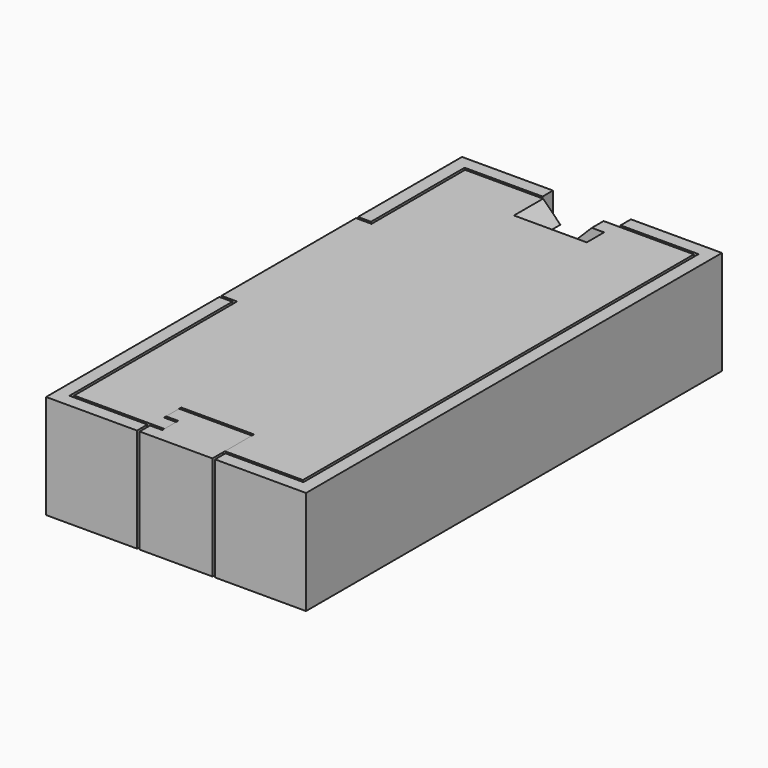
from build123d import *

# Parameters (mm, degrees)
F0_W      = 30
F0_H      = 60
F0_W_2    = 27
F0_H_2    = 57
F0_W_3    = 26.4
F0_H_3    = 56.4
F0_W_4    = 24
F0_H_4    = 54
F1_DEPTH  = 10
F2_DEPTH  = 3
F3_W      = 30
F3_H      = 60
F4_DEPTH  = 2
F6_DEPTH  = 24
F7_DEPTH  = 2
F10_DEPTH = 1.8
F11_DEPTH = 6
F12_START = -3.5
F12_DEPTH = 2.5
F14_DEPTH = 1.8
F15_DEPTH = 6
F16_START = -3.5
F16_DEPTH = 2.5
F17_DEPTH = 6
F18_START = -3.5
F18_DEPTH = 2.5
F19_W     = 8.4
F19_H     = 12
F20_DEPTH = 1.5
F21_DEPTH = 5.7
F22_START = -3.8
F22_DEPTH = 1.9
F23_DEPTH = 6
F24_START = -3.5
F24_DEPTH = 2.5
F25_W     = 20
F25_H     = 8
F26_DEPTH = 3
F27_W     = 3
F27_H     = 19.4
F28_DEPTH = 4
F30_DEPTH = 4.2


with BuildPart() as f1:
    # F0 (on Top) → F1 (new body)
    with BuildSketch(Plane.XY):
        with Locations((15, 30)):
            Rectangle(F0_W, F0_H)
        with Locations((15, 30)):
            Rectangle(F0_W_2, F0_H_2, mode=Mode.SUBTRACT)
        with Locations((15, 30)):
            Rectangle(F0_W_2, F0_H_2)
        with Locations((15, 30)):
            Rectangle(F0_W_3, F0_H_3, mode=Mode.SUBTRACT)
        with Locations((15, 30)):
            Rectangle(F0_W_3, F0_H_3)
        with Locations((15, 30)):
            Rectangle(F0_W_4, F0_H_4, mode=Mode.SUBTRACT)
    extrude(amount=-F1_DEPTH)

    # F0 (on Top) → F2 (cut)
    with BuildSketch(Plane.XY):
        with Locations((15, 30)):
            Rectangle(F0_W_2, F0_H_2)
        with Locations((15, 30)):
            Rectangle(F0_W_3, F0_H_3, mode=Mode.SUBTRACT)
        with Locations((15, 30)):
            Rectangle(F0_W_3, F0_H_3)
        with Locations((15, 30)):
            Rectangle(F0_W_4, F0_H_4, mode=Mode.SUBTRACT)
    extrude(amount=-F2_DEPTH, mode=Mode.SUBTRACT)

    # F3 (on face) → F4 (join)
    with BuildSketch(Plane(origin=(0, 0, -10), x_dir=(1, 0, 0), z_dir=(0, 0, -1))):
        with Locations((15, -30)):
            Rectangle(F3_W, F3_H)
    extrude(amount=F4_DEPTH)

    # F5 (on face) → F6 (join, through all)
    with BuildSketch(Plane(origin=(27, 0, 0), x_dir=(0, -1, 0), z_dir=(-1, 0, 0))):
        Polygon((-8, -5), (-3, -10), (-3, -5), align=None)
        Polygon((-57, -5), (-57, -10), (-52, -5), align=None)
    extrude(amount=F6_DEPTH)

    # F9 (on face) → F10 (cut, through all)
    with BuildSketch(Plane.XZ):
        Polygon((10.8, 0), (10.5, 0), (10.5, -12), (10.8, -12), (15, -7.8), (15.7071067812, -8.5071067812), (19.2, -12), (19.5, -12), (19.5, 0), (19.2, 0), (17.2, -2), (14.2142135624, -2), (12.8, -2), align=None)
        Polygon((12.2142135624, 0), (10.8, 0), (12.8, -2), (14.2142135624, -2), align=None)
        Polygon((19.2, 0), (12.2142135624, 0), (14.2142135624, -2), (17.2, -2), align=None)
        Polygon((15.7071067812, -8.5071067812), (12.2142135624, -12), (19.2, -12), align=None)
        Polygon((15, -7.8), (10.8, -12), (12.2142135624, -12), (15.7071067812, -8.5071067812), align=None)
    extrude(amount=-F10_DEPTH, mode=Mode.SUBTRACT)

    # F13 (on face) → F14 (cut, through all)
    with BuildSketch(Plane(origin=(0, 60, 0), x_dir=(-1, 0, 0), z_dir=(0, 1, 0))):
        Polygon((-19.2, 0), (-19.5, 0), (-19.5, -12), (-19.2, -12), (-15, -7.8), (-14.2928932188, -8.5071067812), (-10.8, -12), (-10.5, -12), (-10.5, 0), (-10.8, 0), (-12.8, -2), (-15.7857864376, -2), (-17.2, -2), align=None)
        Polygon((-17.7857864376, 0), (-19.2, 0), (-17.2, -2), (-15.7857864376, -2), align=None)
        Polygon((-10.8, 0), (-17.7857864376, 0), (-15.7857864376, -2), (-12.8, -2), align=None)
        Polygon((-14.2928932188, -8.5071067812), (-17.7857864376, -12), (-10.8, -12), align=None)
        Polygon((-15, -7.8), (-19.2, -12), (-17.7857864376, -12), (-14.2928932188, -8.5071067812), align=None)
    extrude(amount=-F14_DEPTH, mode=Mode.SUBTRACT)

    # F9 (on face) → F17 (cut)
    with BuildSketch(Plane.XZ):
        Polygon((15.7071067812, -8.5071067812), (12.2142135624, -12), (19.2, -12), align=None)
    extrude(amount=-F17_DEPTH, mode=Mode.SUBTRACT)

    # F9 (on face) → F18 (cut)
    with BuildSketch(Plane.XZ.offset(F18_START)):
        Polygon((15, -7.8), (10.8, -12), (12.2142135624, -12), (15.7071067812, -8.5071067812), align=None)
    extrude(amount=-F18_DEPTH, mode=Mode.SUBTRACT)

    # F13 (on face) → F23 (cut)
    with BuildSketch(Plane(origin=(0, 60, 0), x_dir=(-1, 0, 0), z_dir=(0, 1, 0))):
        Polygon((-14.2928932188, -8.5071067812), (-17.7857864376, -12), (-10.8, -12), align=None)
    extrude(amount=-F23_DEPTH, mode=Mode.SUBTRACT)

    # F13 (on face) → F24 (cut)
    with BuildSketch(Plane(origin=(0, 60, 0), x_dir=(-1, 0, 0), z_dir=(0, 1, 0)).offset(F24_START)):
        Polygon((-15, -7.8), (-19.2, -12), (-17.7857864376, -12), (-14.2928932188, -8.5071067812), align=None)
    extrude(amount=-F24_DEPTH, mode=Mode.SUBTRACT)

    # F25 (on face) → F26 (cut, through all)
    with BuildSketch(Plane(origin=(0, 0, 0), x_dir=(0, -1, 0), z_dir=(-1, 0, 0))):
        with Locations((-35, -4)):
            Rectangle(F25_W, F25_H)
    extrude(amount=-F26_DEPTH, mode=Mode.SUBTRACT)


with BuildPart() as f7:
    # F0 (on Top) → F7 (new body)
    with BuildSketch(Plane.XY):
        with Locations((15, 30)):
            Rectangle(F0_W_3, F0_H_3)
        with Locations((15, 30)):
            Rectangle(F0_W_4, F0_H_4, mode=Mode.SUBTRACT)
        with Locations((15, 30)):
            Rectangle(F0_W_4, F0_H_4)
    extrude(amount=-F7_DEPTH)

    # F9 (on face) → F11 (cut)
    with BuildSketch(Plane.XZ):
        Polygon((19.2, 0), (12.2142135624, 0), (14.2142135624, -2), (17.2, -2), align=None)
    extrude(amount=-F11_DEPTH, mode=Mode.SUBTRACT)

    # F9 (on face) → F12 (cut)
    with BuildSketch(Plane.XZ.offset(F12_START)):
        Polygon((12.2142135624, 0), (10.8, 0), (12.8, -2), (14.2142135624, -2), align=None)
    extrude(amount=-F12_DEPTH, mode=Mode.SUBTRACT)

    # F13 (on face) → F15 (cut)
    with BuildSketch(Plane(origin=(0, 60, 0), x_dir=(-1, 0, 0), z_dir=(0, 1, 0))):
        Polygon((-10.8, 0), (-17.7857864376, 0), (-15.7857864376, -2), (-12.8, -2), align=None)
    extrude(amount=-F15_DEPTH, mode=Mode.SUBTRACT)

    # F13 (on face) → F16 (cut)
    with BuildSketch(Plane(origin=(0, 60, 0), x_dir=(-1, 0, 0), z_dir=(0, 1, 0)).offset(F16_START)):
        Polygon((-17.7857864376, 0), (-19.2, 0), (-17.2, -2), (-15.7857864376, -2), align=None)
    extrude(amount=-F16_DEPTH, mode=Mode.SUBTRACT)

    # F27 (on face) → F28 (join)
    with BuildSketch(Plane.XY):
        with Locations((1.5, 35)):
            Rectangle(F27_W, F27_H)
    extrude(amount=-F28_DEPTH)


with BuildPart() as f20:
    # F19 (on face) → F20 (new body)
    with BuildSketch(Plane.XZ):
        with Locations((15, -6)):
            Rectangle(F19_W, F19_H)
    extrude(amount=-F20_DEPTH)

    # F9 (on face) → F21 (join)
    with BuildSketch(Plane.XZ):
        Polygon((19.2, 0), (12.2142135624, 0), (14.2142135624, -2), (17.2, -2), align=None)
        Polygon((15.7071067812, -8.5071067812), (12.2142135624, -12), (19.2, -12), align=None)
    extrude(amount=-F21_DEPTH)

    # F9 (on face) → F22 (join)
    with BuildSketch(Plane.XZ.offset(F22_START)):
        Polygon((12.2142135624, 0), (10.8, 0), (12.8, -2), (14.2142135624, -2), align=None)
        Polygon((15, -7.8), (10.8, -12), (12.2142135624, -12), (15.7071067812, -8.5071067812), align=None)
    extrude(amount=-F22_DEPTH)

    # F29 (on face) → F30 (cut, through all)
    with BuildSketch(Plane(origin=(0, 5.7, 0), x_dir=(-1, 0, 0), z_dir=(0, 1, 0))):
        Polygon((-12.8, -10), (-15, -7.8), (-17.2, -10), align=None)
    extrude(amount=-F30_DEPTH, mode=Mode.SUBTRACT)


solid = Compound([f1.part, f7.part, f20.part])
